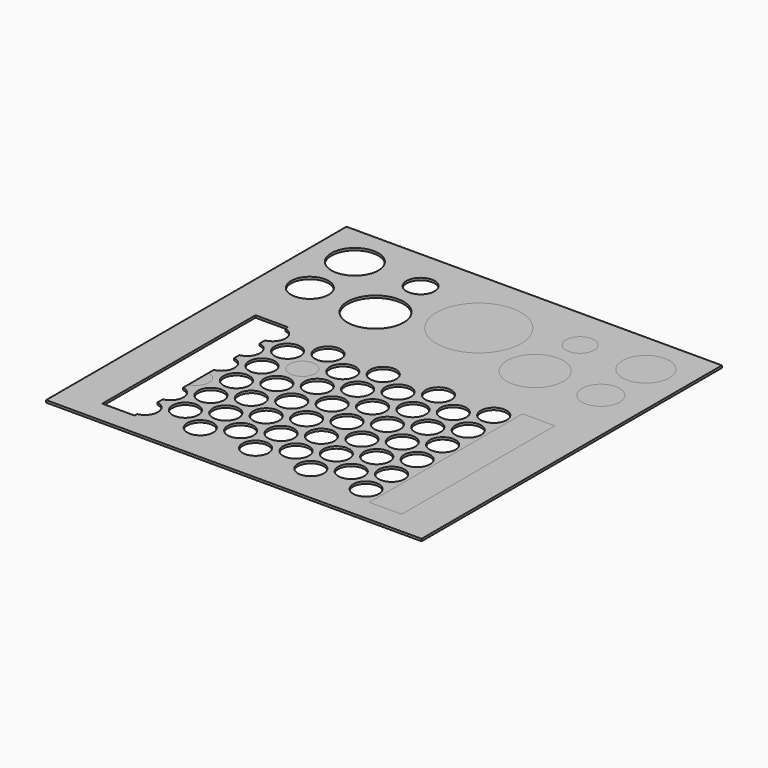
from build123d import *

# Parameters (mm, degrees)
F0_W     = 50.8
F0_H     = 50.8
F0_R     = 2.54
F0_R_2   = 3.81
F0_R_3   = 3.175
F0_R_4   = 5.715
F0_R_5   = 1.905
F0_R_6   = 1.7526
F1_DEPTH = 0.3048
F2_DEPTH = 0.3048


# Not quite as in the source:
# - a feature names something its author has since deleted; it is built from what else it names


with BuildPart() as f1:
    # F0 (on Top) → F1 (new body)
    with BuildSketch(Plane.XY):
        with Locations((0, 9.3726)):
            Rectangle(F0_W, F0_H)
        with BuildLine():
            Line((-15.875, -12.954), (-20.2565, -12.954))
            Line((-20.2565, -12.954), (-20.2565, 12.954))
            Line((-20.2565, 12.954), (-15.875, 12.954))
            Line((-15.875, 12.954), (-14.2175923118, 12.954))
            ThreePointArc((-14.2175923118, 12.954), (-12.4649923118, 14.7066), (-10.7123923118, 12.954))
            Line((-10.7123923118, 12.954), (-6.7385969247, 12.954))
            ThreePointArc((-6.7385969247, 12.954), (-4.9859969247, 14.7066), (-3.2333969247, 12.954))
            Line((-3.2333969247, 12.954), (0.7403984624, 12.954))
            ThreePointArc((0.7403984624, 12.954), (2.4929984624, 14.7066), (4.2455984624, 12.954))
            Line((4.2455984624, 12.954), (8.2193938494, 12.954))
            ThreePointArc((8.2193938494, 12.954), (9.9719938494, 14.7066), (11.7245938494, 12.954))
            Line((11.7245938494, 12.954), (15.6983892365, 12.954))
            ThreePointArc((15.6983892365, 12.954), (17.4509892365, 14.7066), (19.2035892365, 12.954))
            Line((19.2035892365, 12.954), (20.2565, 12.954))
            Line((20.2565, 12.954), (20.2565, -12.954))
            Line((20.2565, -12.954), (15.875, -12.954))
            Line((15.875, -12.954), (11.7245938494, -12.954))
            ThreePointArc((11.7245938494, -12.954), (9.9719938494, -14.7066), (8.2193938494, -12.954))
            Line((8.2193938494, -12.954), (4.2455984624, -12.954))
            ThreePointArc((4.2455984624, -12.954), (2.4929984624, -14.7066), (0.7403984624, -12.954))
            Line((0.7403984624, -12.954), (-3.2333969247, -12.954))
            ThreePointArc((-3.2333969247, -12.954), (-4.9859969247, -14.7066), (-6.7385969247, -12.954))
            Line((-6.7385969247, -12.954), (-10.7123923118, -12.954))
            ThreePointArc((-10.7123923118, -12.954), (-12.4649923118, -14.7066), (-14.2175923118, -12.954))
            Line((-14.2175923118, -12.954), (-15.875, -12.954))
        make_face(mode=Mode.SUBTRACT)
        with Locations((-19.685, 21.4376)):
            Circle(F0_R, mode=Mode.SUBTRACT)
        with Locations((-10.795, 21.4376)):
            Circle(F0_R_2, mode=Mode.SUBTRACT)
        with Locations((-19.685, 29.0576)):
            Circle(F0_R_3, mode=Mode.SUBTRACT)
        with Locations((0, 25.4)):
            Circle(F0_R_4, mode=Mode.SUBTRACT)
        with Locations((-10.795, 29.0576)):
            Circle(F0_R_5, mode=Mode.SUBTRACT)
        with Locations((10.795, 21.4376)):
            Circle(F0_R_2, mode=Mode.SUBTRACT)
        with Locations((19.685, 21.4376)):
            Circle(F0_R, mode=Mode.SUBTRACT)
        with Locations((10.795, 29.0576)):
            Circle(F0_R_5, mode=Mode.SUBTRACT)
        with Locations((19.685, 29.0576)):
            Circle(F0_R_3, mode=Mode.SUBTRACT)
        with BuildLine():
            ThreePointArc((-10.7123923118, 12.954), (-12.4649923118, 14.7066), (-14.2175923118, 12.954))
            Line((-14.2175923118, 12.954), (-10.7123923118, 12.954))
        make_face()
        with BuildLine():
            ThreePointArc((-3.2333969247, 12.954), (-4.9859969247, 14.7066), (-6.7385969247, 12.954))
            Line((-6.7385969247, 12.954), (-3.2333969247, 12.954))
        make_face()
        with BuildLine():
            ThreePointArc((4.2455984624, 12.954), (2.4929984624, 14.7066), (0.7403984624, 12.954))
            Line((0.7403984624, 12.954), (4.2455984624, 12.954))
        make_face()
        with BuildLine():
            Line((-3.2333969247, -12.954), (-6.7385969247, -12.954))
            ThreePointArc((-6.7385969247, -12.954), (-4.9859969247, -14.7066), (-3.2333969247, -12.954))
        make_face()
        with BuildLine():
            Line((4.2455984624, -12.954), (0.7403984624, -12.954))
            ThreePointArc((0.7403984624, -12.954), (2.4929984624, -14.7066), (4.2455984624, -12.954))
        make_face()
        with BuildLine():
            Line((11.7245938494, -12.954), (8.2193938494, -12.954))
            ThreePointArc((8.2193938494, -12.954), (9.9719938494, -14.7066), (11.7245938494, -12.954))
        make_face()
        with BuildLine():
            ThreePointArc((11.7245938494, 12.954), (9.9719938494, 14.7066), (8.2193938494, 12.954))
            Line((8.2193938494, 12.954), (11.7245938494, 12.954))
        make_face()
        with BuildLine():
            Line((-10.7123923118, -12.954), (-14.2175923118, -12.954))
            ThreePointArc((-14.2175923118, -12.954), (-12.4649923118, -14.7066), (-10.7123923118, -12.954))
        make_face()
        with BuildLine():
            Line((-15.875, -12.5163492081), (-15.875, -12.954))
            Line((-15.875, -12.954), (-14.2175923118, -12.954))
            ThreePointArc((-14.2175923118, -12.954), (-12.4649923118, -11.2014), (-10.7123923118, -12.954))
            Line((-10.7123923118, -12.954), (-6.7385969247, -12.954))
            ThreePointArc((-6.7385969247, -12.954), (-4.9859969247, -11.2014), (-3.2333969247, -12.954))
            Line((-3.2333969247, -12.954), (0.7403984624, -12.954))
            ThreePointArc((0.7403984624, -12.954), (2.4929984624, -11.2014), (4.2455984624, -12.954))
            Line((4.2455984624, -12.954), (8.2193938494, -12.954))
            ThreePointArc((8.2193938494, -12.954), (9.9719938494, -11.2014), (11.7245938494, -12.954))
            Line((11.7245938494, -12.954), (15.875, -12.954))
            Line((15.875, -12.954), (15.875, -9.4027233441))
            ThreePointArc((15.875, -9.4027233441), (15.6983892365, -8.636), (15.875, -7.8692766559))
            Line((15.875, -7.8692766559), (15.875, -5.0847233441))
            ThreePointArc((15.875, -5.0847233441), (15.6983892365, -4.318), (15.875, -3.5512766559))
            Line((15.875, -3.5512766559), (15.875, -0.7667233441))
            ThreePointArc((15.875, -0.7667233441), (15.6983892365, 0), (15.875, 0.7667233441))
            Line((15.875, 0.7667233441), (15.875, 3.5512766559))
            ThreePointArc((15.875, 3.5512766559), (15.6983892365, 4.318), (15.875, 5.0847233441))
            Line((15.875, 5.0847233441), (15.875, 7.8692766559))
            ThreePointArc((15.875, 7.8692766559), (15.6983892365, 8.636), (15.875, 9.4027233441))
            Line((15.875, 9.4027233441), (15.875, 12.1872766559))
            ThreePointArc((15.875, 12.1872766559), (15.7431125583, 12.5605994255), (15.6983892365, 12.954))
            Line((15.6983892365, 12.954), (11.7245938494, 12.954))
            ThreePointArc((11.7245938494, 12.954), (9.9719938494, 11.2014), (8.2193938494, 12.954))
            Line((8.2193938494, 12.954), (4.2455984624, 12.954))
            ThreePointArc((4.2455984624, 12.954), (2.4929984624, 11.2014), (0.7403984624, 12.954))
            Line((0.7403984624, 12.954), (-3.2333969247, 12.954))
            ThreePointArc((-3.2333969247, 12.954), (-4.9859969247, 11.2014), (-6.7385969247, 12.954))
            Line((-6.7385969247, 12.954), (-10.7123923118, 12.954))
            ThreePointArc((-10.7123923118, 12.954), (-12.4649923118, 11.2014), (-14.2175923118, 12.954))
            Line((-14.2175923118, 12.954), (-15.875, 12.954))
            Line((-15.875, 12.954), (-15.875, 12.5163492081))
            ThreePointArc((-15.875, 12.5163492081), (-14.8537363373, 11.911723461), (-14.4518900053, 10.795))
            ThreePointArc((-14.4518900053, 10.795), (-14.8537363373, 9.678276539), (-15.875, 9.0736507919))
            Line((-15.875, 9.0736507919), (-15.875, 8.1983492081))
            ThreePointArc((-15.875, 8.1983492081), (-14.8537363373, 7.593723461), (-14.4518900053, 6.477))
            ThreePointArc((-14.4518900053, 6.477), (-14.8537363373, 5.360276539), (-15.875, 4.7556507919))
            Line((-15.875, 4.7556507919), (-15.875, 3.8803492081))
            ThreePointArc((-15.875, 3.8803492081), (-14.8537363373, 3.275723461), (-14.4518900053, 2.159))
            ThreePointArc((-14.4518900053, 2.159), (-14.8537363373, 1.042276539), (-15.875, 0.4376507919))
            Line((-15.875, 0.4376507919), (-15.875, -0.4376507919))
            ThreePointArc((-15.875, -0.4376507919), (-14.8537363373, -1.042276539), (-14.4518900053, -2.159))
            ThreePointArc((-14.4518900053, -2.159), (-14.8537363373, -3.275723461), (-15.875, -3.8803492081))
            Line((-15.875, -3.8803492081), (-15.875, -4.7556507919))
            ThreePointArc((-15.875, -4.7556507919), (-14.8537363373, -5.360276539), (-14.4518900053, -6.477))
            ThreePointArc((-14.4518900053, -6.477), (-14.8537363373, -7.593723461), (-15.875, -8.1983492081))
            Line((-15.875, -8.1983492081), (-15.875, -9.0736507919))
            ThreePointArc((-15.875, -9.0736507919), (-14.8537363373, -9.678276539), (-14.4518900053, -10.795))
            ThreePointArc((-14.4518900053, -10.795), (-14.8537363373, -11.911723461), (-15.875, -12.5163492081))
        make_face()
        with Locations((-8.7254946183, -10.795)):
            Circle(F0_R_6, mode=Mode.SUBTRACT)
        with Locations((-1.2464992312, -10.795)):
            Circle(F0_R_6, mode=Mode.SUBTRACT)
        with Locations((-12.4649923118, -8.636)):
            Circle(F0_R_6, mode=Mode.SUBTRACT)
        with Locations((-12.4649923118, -4.318)):
            Circle(F0_R_6, mode=Mode.SUBTRACT)
        with Locations((-8.7254946183, -6.477)):
            Circle(F0_R_6, mode=Mode.SUBTRACT)
        with Locations((-4.9859969247, -8.636)):
            Circle(F0_R_6, mode=Mode.SUBTRACT)
        with Locations((-4.9859969247, -4.318)):
            Circle(F0_R_6, mode=Mode.SUBTRACT)
        with Locations((-1.2464992312, -6.477)):
            Circle(F0_R_6, mode=Mode.SUBTRACT)
        with Locations((-8.7254946183, -2.159)):
            Circle(F0_R_6, mode=Mode.SUBTRACT)
        with Locations((-12.4649923118, 0)):
            Circle(F0_R_6, mode=Mode.SUBTRACT)
        with Locations((-8.7254946183, 2.159)):
            Circle(F0_R_6, mode=Mode.SUBTRACT)
        with Locations((-1.2464992312, -2.159)):
            Circle(F0_R_6, mode=Mode.SUBTRACT)
        with Locations((-4.9859969247, 0)):
            Circle(F0_R_6, mode=Mode.SUBTRACT)
        with Locations((-1.2464992312, 2.159)):
            Circle(F0_R_6, mode=Mode.SUBTRACT)
        with Locations((-12.4649923118, 4.318)):
            Circle(F0_R_6, mode=Mode.SUBTRACT)
        with Locations((-12.4649923118, 8.636)):
            Circle(F0_R_6, mode=Mode.SUBTRACT)
        with Locations((-8.7254946183, 6.477)):
            Circle(F0_R_6, mode=Mode.SUBTRACT)
        with Locations((-4.9859969247, 4.318)):
            Circle(F0_R_6, mode=Mode.SUBTRACT)
        with Locations((-4.9859969247, 8.636)):
            Circle(F0_R_6, mode=Mode.SUBTRACT)
        with Locations((-1.2464992312, 6.477)):
            Circle(F0_R_6, mode=Mode.SUBTRACT)
        with Locations((6.2324961559, -10.795)):
            Circle(F0_R_6, mode=Mode.SUBTRACT)
        with Locations((2.4929984624, -8.636)):
            Circle(F0_R_6, mode=Mode.SUBTRACT)
        with Locations((2.4929984624, -4.318)):
            Circle(F0_R_6, mode=Mode.SUBTRACT)
        with Locations((6.2324961559, -6.477)):
            Circle(F0_R_6, mode=Mode.SUBTRACT)
        with Locations((9.9719938494, -8.636)):
            Circle(F0_R_6, mode=Mode.SUBTRACT)
        with Locations((9.9719938494, -4.318)):
            Circle(F0_R_6, mode=Mode.SUBTRACT)
        with Locations((13.711491543, -10.795)):
            Circle(F0_R_6, mode=Mode.SUBTRACT)
        with Locations((13.711491543, -6.477)):
            Circle(F0_R_6, mode=Mode.SUBTRACT)
        with Locations((6.2324961559, -2.159)):
            Circle(F0_R_6, mode=Mode.SUBTRACT)
        with Locations((2.4929984624, 0)):
            Circle(F0_R_6, mode=Mode.SUBTRACT)
        with Locations((6.2324961559, 2.159)):
            Circle(F0_R_6, mode=Mode.SUBTRACT)
        with Locations((9.9719938494, 0)):
            Circle(F0_R_6, mode=Mode.SUBTRACT)
        with Locations((2.4929984624, 4.318)):
            Circle(F0_R_6, mode=Mode.SUBTRACT)
        with Locations((2.4929984624, 8.636)):
            Circle(F0_R_6, mode=Mode.SUBTRACT)
        with Locations((6.2324961559, 6.477)):
            Circle(F0_R_6, mode=Mode.SUBTRACT)
        with Locations((9.9719938494, 4.318)):
            Circle(F0_R_6, mode=Mode.SUBTRACT)
        with Locations((9.9719938494, 8.636)):
            Circle(F0_R_6, mode=Mode.SUBTRACT)
        with Locations((13.711491543, -2.159)):
            Circle(F0_R_6, mode=Mode.SUBTRACT)
        with Locations((13.711491543, 2.159)):
            Circle(F0_R_6, mode=Mode.SUBTRACT)
        with Locations((13.711491543, 6.477)):
            Circle(F0_R_6, mode=Mode.SUBTRACT)
        with Locations((-8.7254946183, 10.795)):
            Circle(F0_R_6, mode=Mode.SUBTRACT)
        with Locations((-1.2464992312, 10.795)):
            Circle(F0_R_6, mode=Mode.SUBTRACT)
        with Locations((6.2324961559, 10.795)):
            Circle(F0_R_6, mode=Mode.SUBTRACT)
        with Locations((13.711491543, 10.795)):
            Circle(F0_R_6, mode=Mode.SUBTRACT)
        with BuildLine():
            ThreePointArc((19.2035892365, 12.954), (17.4509892365, 14.7066), (15.6983892365, 12.954))
            Line((15.6983892365, 12.954), (15.875, 12.954))
            Line((15.875, 12.954), (19.2035892365, 12.954))
        make_face()
        with BuildLine():
            ThreePointArc((15.875, -3.5512766559), (15.6983892365, -4.318), (15.875, -5.0847233441))
            Line((15.875, -5.0847233441), (15.875, -3.5512766559))
        make_face()
        with BuildLine():
            ThreePointArc((15.875, -7.8692766559), (15.6983892365, -8.636), (15.875, -9.4027233441))
            Line((15.875, -9.4027233441), (15.875, -7.8692766559))
        make_face()
        with BuildLine():
            ThreePointArc((15.875, 0.7667233441), (15.6983892365, 0), (15.875, -0.7667233441))
            Line((15.875, -0.7667233441), (15.875, 0.7667233441))
        make_face()
        with BuildLine():
            Line((15.875, 3.5512766559), (15.875, 5.0847233441))
            ThreePointArc((15.875, 5.0847233441), (15.6983892365, 4.318), (15.875, 3.5512766559))
        make_face()
        with BuildLine():
            Line((15.875, 7.8692766559), (15.875, 9.4027233441))
            ThreePointArc((15.875, 9.4027233441), (15.6983892365, 8.636), (15.875, 7.8692766559))
        make_face()
        with BuildLine():
            Line((15.875, 12.954), (15.6983892365, 12.954))
            ThreePointArc((15.6983892365, 12.954), (15.7431125583, 12.5605994255), (15.875, 12.1872766559))
            Line((15.875, 12.1872766559), (15.875, 12.954))
        make_face()
        with BuildLine():
            Line((-10.7123923118, 12.954), (-14.2175923118, 12.954))
            ThreePointArc((-14.2175923118, 12.954), (-12.4649923118, 11.2014), (-10.7123923118, 12.954))
        make_face()
        with BuildLine():
            Line((-3.2333969247, 12.954), (-6.7385969247, 12.954))
            ThreePointArc((-6.7385969247, 12.954), (-4.9859969247, 11.2014), (-3.2333969247, 12.954))
        make_face()
        with BuildLine():
            Line((4.2455984624, 12.954), (0.7403984624, 12.954))
            ThreePointArc((0.7403984624, 12.954), (2.4929984624, 11.2014), (4.2455984624, 12.954))
        make_face()
        with BuildLine():
            Line((11.7245938494, 12.954), (8.2193938494, 12.954))
            ThreePointArc((8.2193938494, 12.954), (9.9719938494, 11.2014), (11.7245938494, 12.954))
        make_face()
        with BuildLine():
            ThreePointArc((11.7245938494, -12.954), (9.9719938494, -11.2014), (8.2193938494, -12.954))
            Line((8.2193938494, -12.954), (11.7245938494, -12.954))
        make_face()
        with BuildLine():
            ThreePointArc((4.2455984624, -12.954), (2.4929984624, -11.2014), (0.7403984624, -12.954))
            Line((0.7403984624, -12.954), (4.2455984624, -12.954))
        make_face()
        with BuildLine():
            ThreePointArc((-3.2333969247, -12.954), (-4.9859969247, -11.2014), (-6.7385969247, -12.954))
            Line((-6.7385969247, -12.954), (-3.2333969247, -12.954))
        make_face()
        with BuildLine():
            ThreePointArc((-10.7123923118, -12.954), (-12.4649923118, -11.2014), (-14.2175923118, -12.954))
            Line((-14.2175923118, -12.954), (-10.7123923118, -12.954))
        make_face()
    extrude(amount=F1_DEPTH)


with BuildPart() as f2:
    # F0 (on Top) → F2 (new body)
    with BuildSketch(Plane.XY):
        with Locations((0, 25.4)):
            Circle(F0_R_4)
    extrude(amount=F2_DEPTH)


with BuildPart() as f2b:
    # F0 (on Top) → F2, piece 2 (new body)
    with BuildSketch(Plane.XY):
        with Locations((10.795, 21.4376)):
            Circle(F0_R_2)
    extrude(amount=F2_DEPTH)


with BuildPart() as f2c:
    # F0 (on Top) → F2, piece 3 (new body)
    with BuildSketch(Plane.XY):
        with Locations((10.795, 29.0576)):
            Circle(F0_R_5)
    extrude(amount=F2_DEPTH)


with BuildPart() as f2d:
    # F0 (on Top) → F2, piece 4 (new body)
    with BuildSketch(Plane.XY):
        with Locations((19.685, 29.0576)):
            Circle(F0_R_3)
    extrude(amount=F2_DEPTH)


with BuildPart() as f2e:
    # F0 (on Top) → F2, piece 5 (new body)
    with BuildSketch(Plane.XY):
        with Locations((19.685, 21.4376)):
            Circle(F0_R)
    extrude(amount=F2_DEPTH)


with BuildPart() as f2f:
    # F0 (on Top) → F2, piece 6 (new body)
    with BuildSketch(Plane.XY):
        with Locations((-8.7254946183, 6.477)):
            Circle(F0_R_6)
    extrude(amount=F2_DEPTH)


with BuildPart() as f2g:
    # F0 (on Top) → F2, piece 7 (new body)
    with BuildSketch(Plane.XY):
        with BuildLine():
            Line((-3.2333969247, 12.954), (-6.7385969247, 12.954))
            ThreePointArc((-6.7385969247, 12.954), (-4.9859969247, 11.2014), (-3.2333969247, 12.954))
        make_face()
    extrude(amount=F2_DEPTH)


with BuildPart() as f2h:
    # F0 (on Top) → F2, piece 8 (new body)
    with BuildSketch(Plane.XY):
        with BuildLine():
            Line((15.875, -9.4027233441), (15.875, -12.954))
            Line((15.875, -12.954), (20.2565, -12.954))
            Line((20.2565, -12.954), (20.2565, 12.954))
            Line((20.2565, 12.954), (19.2035892365, 12.954))
            ThreePointArc((19.2035892365, 12.954), (17.844389811, 11.2461233218), (15.875, 12.1872766559))
            Line((15.875, 12.1872766559), (15.875, 9.4027233441))
            ThreePointArc((15.875, 9.4027233441), (17.844389811, 10.3438766782), (19.2035892365, 8.636))
            ThreePointArc((19.2035892365, 8.636), (17.844389811, 6.9281233218), (15.875, 7.8692766559))
            Line((15.875, 7.8692766559), (15.875, 5.0847233441))
            ThreePointArc((15.875, 5.0847233441), (17.844389811, 6.0258766782), (19.2035892365, 4.318))
            ThreePointArc((19.2035892365, 4.318), (17.844389811, 2.6101233218), (15.875, 3.5512766559))
            Line((15.875, 3.5512766559), (15.875, 0.7667233441))
            ThreePointArc((15.875, 0.7667233441), (17.844389811, 1.7078766782), (19.2035892365, 0))
            ThreePointArc((19.2035892365, 0), (17.844389811, -1.7078766782), (15.875, -0.7667233441))
            Line((15.875, -0.7667233441), (15.875, -3.5512766559))
            ThreePointArc((15.875, -3.5512766559), (17.844389811, -2.6101233218), (19.2035892365, -4.318))
            ThreePointArc((19.2035892365, -4.318), (17.844389811, -6.0258766782), (15.875, -5.0847233441))
            Line((15.875, -5.0847233441), (15.875, -7.8692766559))
            ThreePointArc((15.875, -7.8692766559), (17.844389811, -6.9281233218), (19.2035892365, -8.636))
            ThreePointArc((19.2035892365, -8.636), (17.844389811, -10.3438766782), (15.875, -9.4027233441))
        make_face()
        with BuildLine():
            Line((15.875, 0.7667233441), (15.875, -0.7667233441))
            ThreePointArc((15.875, -0.7667233441), (17.844389811, -1.7078766782), (19.2035892365, 0))
            ThreePointArc((19.2035892365, 0), (17.844389811, 1.7078766782), (15.875, 0.7667233441))
        make_face()
        with BuildLine():
            ThreePointArc((19.2035892365, 4.318), (17.844389811, 6.0258766782), (15.875, 5.0847233441))
            Line((15.875, 5.0847233441), (15.875, 3.5512766559))
            ThreePointArc((15.875, 3.5512766559), (17.844389811, 2.6101233218), (19.2035892365, 4.318))
        make_face()
        with BuildLine():
            ThreePointArc((19.2035892365, 8.636), (17.844389811, 10.3438766782), (15.875, 9.4027233441))
            Line((15.875, 9.4027233441), (15.875, 7.8692766559))
            ThreePointArc((15.875, 7.8692766559), (17.844389811, 6.9281233218), (19.2035892365, 8.636))
        make_face()
        with BuildLine():
            Line((19.2035892365, 12.954), (15.875, 12.954))
            Line((15.875, 12.954), (15.875, 12.1872766559))
            ThreePointArc((15.875, 12.1872766559), (17.844389811, 11.2461233218), (19.2035892365, 12.954))
        make_face()
        with BuildLine():
            Line((15.875, -3.5512766559), (15.875, -5.0847233441))
            ThreePointArc((15.875, -5.0847233441), (17.844389811, -6.0258766782), (19.2035892365, -4.318))
            ThreePointArc((19.2035892365, -4.318), (17.844389811, -2.6101233218), (15.875, -3.5512766559))
        make_face()
        with BuildLine():
            Line((15.875, -7.8692766559), (15.875, -9.4027233441))
            ThreePointArc((15.875, -9.4027233441), (17.844389811, -10.3438766782), (19.2035892365, -8.636))
            ThreePointArc((19.2035892365, -8.636), (17.844389811, -6.9281233218), (15.875, -7.8692766559))
        make_face()
    extrude(amount=F2_DEPTH)


with BuildPart() as f2i:
    # F0 (on Top) → F2, piece 9 (new body)
    with BuildSketch(Plane.XY):
        with BuildLine():
            Line((-15.875, -0.4376507919), (-15.875, -3.8803492081))
            ThreePointArc((-15.875, -3.8803492081), (-14.8537363373, -3.275723461), (-14.4518900053, -2.159))
            ThreePointArc((-14.4518900053, -2.159), (-14.8537363373, -1.042276539), (-15.875, -0.4376507919))
        make_face()
    extrude(amount=F2_DEPTH)


solid = Compound([f1.part, f2.part, f2b.part, f2c.part, f2d.part, f2e.part, f2f.part, f2h.part, f2i.part])
